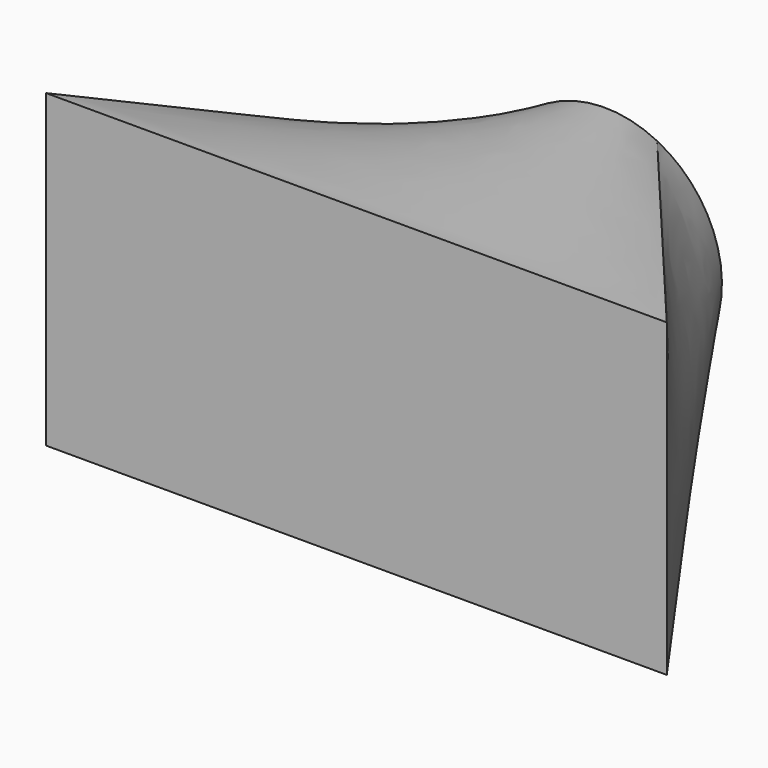
from build123d import *

# Parameters (mm, degrees)
F0_W = 100
F0_H = 50


# Not quite as in the source:
# - the arcs of a loft's sections are written as splines that run evenly, so that the points pair up as in the source's solid


with BuildPart() as f3:
    # F0 (on Front) → F3 section 0
    with BuildSketch(Plane.XZ):
        Rectangle(F0_W, F0_H)
    # F2 (on offset) → F3 section 1
    with BuildSketch(Plane.XZ.offset(-50)):
        with BuildLine():
            add(Edge.make_bspline(
                [(-16.8978941877, 8.4489470939), (-17.4508764819, 7.3429825055), (-17.8949197916, 6.1825826088), (-18.5481076052, 3.7973920433), (-18.7572359577, 2.572660353), (-18.932545355, 0.1058699345), (-18.898722065, -1.1361277974), (-18.5894160044, -3.5897206965), (-18.313940882, -4.8012551937), (-17.5319058218, -7.1473603742), (-17.0253652214, -8.2818730455), (-15.8006543305, -10.4303310011), (-15.0825143233, -11.4442231607), (-13.4621925543, -13.312469857), (-12.5600508581, -14.1667781978), (-10.606386268, -15.6830179621), (-9.5549116822, -16.3449118936), (-8.4489470939, -16.8978941877)],
                knots=[0, 0, 0, 0, 0.125, 0.125, 0.25, 0.25, 0.375, 0.375, 0.5, 0.5, 0.625, 0.625, 0.75, 0.75, 0.875, 0.875, 1, 1, 1, 1], degree=3))
            add(Edge.make_bspline(
                [(-8.4489470939, -16.8978941877), (-7.3429825055, -17.4508764819), (-6.1825826088, -17.8949197916), (-3.7973920433, -18.5481076052), (-2.572660353, -18.7572359577), (-0.1058699345, -18.932545355), (1.1361277974, -18.898722065), (3.5897206965, -18.5894160044), (4.8012551937, -18.313940882), (7.1473603742, -17.5319058218), (8.2818730455, -17.0253652214), (10.4303310011, -15.8006543305), (11.4442231607, -15.0825143233), (13.312469857, -13.4621925543), (14.1667781978, -12.5600508581), (15.6830179621, -10.606386268), (16.3449118936, -9.5549116822), (16.8978941877, -8.4489470939)],
                knots=[0, 0, 0, 0, 0.125, 0.125, 0.25, 0.25, 0.375, 0.375, 0.5, 0.5, 0.625, 0.625, 0.75, 0.75, 0.875, 0.875, 1, 1, 1, 1], degree=3))
            add(Edge.make_bspline(
                [(16.8978941877, -8.4489470939), (17.4508764819, -7.3429825055), (17.8949197916, -6.1825826088), (18.5481076052, -3.7973920433), (18.7572359577, -2.572660353), (18.932545355, -0.1058699345), (18.898722065, 1.1361277974), (18.5894160044, 3.5897206965), (18.313940882, 4.8012551937), (17.5319058218, 7.1473603742), (17.0253652214, 8.2818730455), (15.8006543305, 10.4303310011), (15.0825143233, 11.4442231607), (13.4621925543, 13.312469857), (12.5600508581, 14.1667781978), (10.606386268, 15.6830179621), (9.5549116822, 16.3449118936), (8.4489470939, 16.8978941877)],
                knots=[0, 0, 0, 0, 0.125, 0.125, 0.25, 0.25, 0.375, 0.375, 0.5, 0.5, 0.625, 0.625, 0.75, 0.75, 0.875, 0.875, 1, 1, 1, 1], degree=3))
            add(Edge.make_bspline(
                [(8.4489470939, 16.8978941877), (7.3429825055, 17.4508764819), (6.1825826088, 17.8949197916), (3.7973920433, 18.5481076052), (2.572660353, 18.7572359577), (0.1058699345, 18.932545355), (-1.1361277974, 18.898722065), (-3.5897206965, 18.5894160044), (-4.8012551937, 18.313940882), (-7.1473603742, 17.5319058218), (-8.2818730455, 17.0253652214), (-10.4303310011, 15.8006543305), (-11.4442231607, 15.0825143233), (-13.312469857, 13.4621925543), (-14.1667781978, 12.5600508581), (-15.6830179621, 10.606386268), (-16.3449118936, 9.5549116822), (-16.8978941877, 8.4489470939)],
                knots=[0, 0, 0, 0, 0.125, 0.125, 0.25, 0.25, 0.375, 0.375, 0.5, 0.5, 0.625, 0.625, 0.75, 0.75, 0.875, 0.875, 1, 1, 1, 1], degree=3))
        make_face()
    loft(ruled=True)


solid = f3.part
